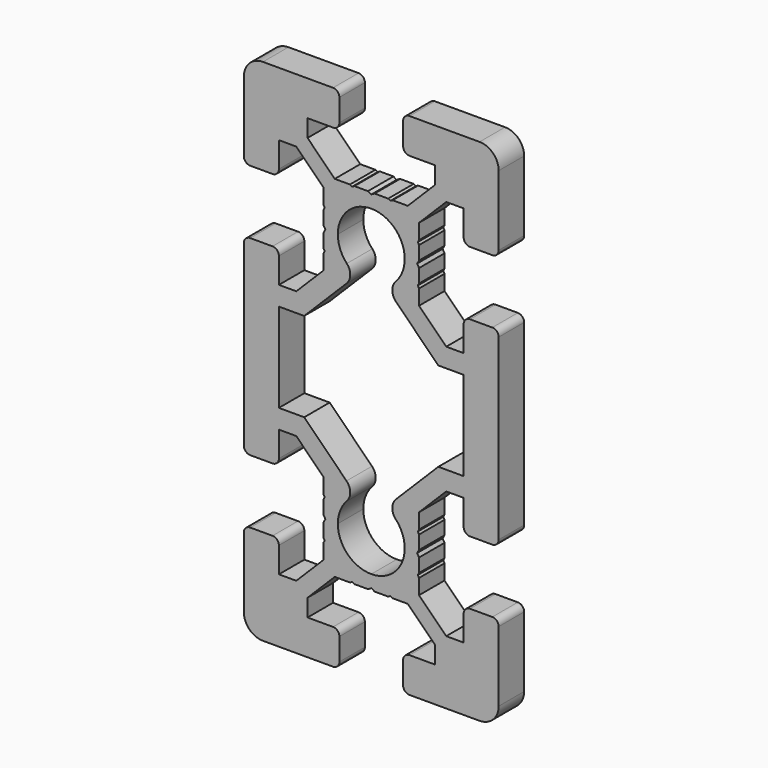
from build123d import *

# Parameters (mm, degrees)
F2_DEPTH = 5


# Not quite as in the source:
# - ends of sketch curves that miss each other by under 0.0002 mm in the source are joined


with BuildPart() as f2:
    # F1 (on Front) → F2 (new body)
    with BuildSketch(Plane.XZ):
        with BuildLine():
            Line((-19.72619, -25.25), (-23.22619, -25.25))
            ThreePointArc((-23.22619, -25.25), (-23.9332967812, -25.5428932188), (-24.22619, -26.25))
            Line((-24.22619, -26.25), (-24.22619, -37.25))
            ThreePointArc((-24.22619, -37.25), (-23.3475103436, -39.3713203436), (-21.22619, -40.25))
            Line((-21.22619, -40.25), (-10.22619, -40.25))
            ThreePointArc((-10.22619, -40.25), (-9.5190832188, -39.9571067812), (-9.22619, -39.25))
            Line((-9.22619, -39.25), (-9.22619, -35.75))
            ThreePointArc((-9.22619, -35.75), (-9.5190832188, -35.0428932188), (-10.22619, -34.75))
            Line((-10.22619, -34.75), (-14.22619, -34.75))
            Line((-14.22619, -34.75), (-14.22619, -32.017775))
            Line((-14.22619, -32.017775), (-9.958438, -27.75))
            Line((-9.958438, -27.75), (-7.5726, -27.75))
            Line((-7.5726, -27.75), (-7.22619, -27.55))
            Line((-7.22619, -27.55), (-6.87978, -27.75))
            Line((-6.87978, -27.75), (-4.745805, -27.75))
            Line((-4.745805, -27.75), (-4.22619, -27.45))
            Line((-4.22619, -27.45), (-3.706575, -27.75))
            Line((-3.706575, -27.75), (-1.5726, -27.75))
            Line((-1.5726, -27.75), (-1.22619, -27.55))
            Line((-1.22619, -27.55), (-0.87978, -27.75))
            Line((-0.87978, -27.75), (1.506057, -27.75))
            Line((1.506057, -27.75), (5.77381, -32.017782))
            Line((5.77381, -32.017782), (5.77381, -34.75))
            Line((5.77381, -34.75), (1.77381, -34.75))
            ThreePointArc((1.77381, -34.75), (1.0667032188, -35.0428932188), (0.77381, -35.75))
            Line((0.77381, -35.75), (0.77381, -39.25))
            ThreePointArc((0.77381, -39.25), (1.0667032188, -39.9571067812), (1.77381, -40.25))
            Line((1.77381, -40.25), (12.77381, -40.25))
            ThreePointArc((12.77381, -40.25), (14.8951303436, -39.3713203436), (15.77381, -37.25))
            Line((15.77381, -37.25), (15.77381, -26.25))
            ThreePointArc((15.77381, -26.25), (15.4809167812, -25.5428932188), (14.77381, -25.25))
            Line((14.77381, -25.25), (11.27381, -25.25))
            ThreePointArc((11.27381, -25.25), (10.5667032188, -25.5428932188), (10.27381, -26.25))
            Line((10.27381, -26.25), (10.27381, -30.25))
            Line((10.27381, -30.25), (7.541595, -30.25))
            Line((7.541595, -30.25), (3.27381, -25.98223))
            Line((3.27381, -25.98223), (3.27381, -23.59641))
            Line((3.27381, -23.59641), (3.07381, -23.25))
            Line((3.07381, -23.25), (3.27381, -22.90359))
            Line((3.27381, -22.90359), (3.27381, -20.769615))
            Line((3.27381, -20.769615), (2.97381, -20.25))
            Line((2.97381, -20.25), (3.27381, -19.730385))
            Line((3.27381, -19.730385), (3.27381, -17.59641))
            Line((3.27381, -17.59641), (3.07381, -17.25))
            Line((3.07381, -17.25), (3.27381, -16.90359))
            Line((3.27381, -16.90359), (3.27381, -14.517762))
            Line((3.27381, -14.517762), (7.541591, -10.25))
            Line((7.541591, -10.25), (10.27381, -10.25))
            Line((10.27381, -10.25), (10.27381, -14.25))
            ThreePointArc((10.27381, -14.25), (10.5667032188, -14.9571067812), (11.27381, -15.25))
            Line((11.27381, -15.25), (14.77381, -15.25))
            ThreePointArc((14.77381, -15.25), (15.4809167812, -14.9571067812), (15.77381, -14.25))
            Line((15.77381, -14.25), (15.77381, 13.75))
            ThreePointArc((15.77381, 13.75), (15.4809167812, 14.4571067812), (14.77381, 14.75))
            Line((14.77381, 14.75), (11.27381, 14.75))
            ThreePointArc((11.27381, 14.75), (10.5667032188, 14.4571067812), (10.27381, 13.75))
            Line((10.27381, 13.75), (10.27381, 9.75))
            Line((10.27381, 9.75), (7.541586, 9.75))
            Line((7.541586, 9.75), (3.27381, 14.01777))
            Line((3.27381, 14.01777), (3.27381, 16.40359))
            Line((3.27381, 16.40359), (3.07381, 16.75))
            Line((3.07381, 16.75), (3.27381, 17.09641))
            Line((3.27381, 17.09641), (3.27381, 19.230385))
            Line((3.27381, 19.230385), (2.97381, 19.75))
            Line((2.97381, 19.75), (3.27381, 20.269615))
            Line((3.27381, 20.269615), (3.27381, 22.40359))
            Line((3.27381, 22.40359), (3.07381, 22.75))
            Line((3.07381, 22.75), (3.27381, 23.09641))
            Line((3.27381, 23.09641), (3.27381, 25.482238))
            Line((3.27381, 25.482238), (7.541577, 29.75))
            Line((7.541577, 29.75), (10.27381, 29.75))
            Line((10.27381, 29.75), (10.27381, 25.75))
            ThreePointArc((10.27381, 25.75), (10.5667032188, 25.0428932188), (11.27381, 24.75))
            Line((11.27381, 24.75), (14.77381, 24.75))
            ThreePointArc((14.77381, 24.75), (15.4809167812, 25.0428932188), (15.77381, 25.75))
            Line((15.77381, 25.75), (15.77381, 36.75))
            ThreePointArc((15.77381, 36.75), (14.8951303436, 38.8713203436), (12.77381, 39.75))
            Line((12.77381, 39.75), (1.77381, 39.75))
            ThreePointArc((1.77381, 39.75), (1.0667032188, 39.4571067812), (0.77381, 38.75))
            Line((0.77381, 38.75), (0.77381, 35.25))
            ThreePointArc((0.77381, 35.25), (1.0667032188, 34.5428932188), (1.77381, 34.25))
            Line((1.77381, 34.25), (5.77381, 34.25))
            Line((5.77381, 34.25), (5.77381, 31.517777))
            Line((5.77381, 31.517777), (1.50604, 27.25))
            Line((1.50604, 27.25), (-0.87978, 27.25))
            Line((-0.87978, 27.25), (-1.22619, 27.05))
            Line((-1.22619, 27.05), (-1.5726, 27.25))
            Line((-1.5726, 27.25), (-3.706575, 27.25))
            Line((-3.706575, 27.25), (-4.22619, 26.95))
            Line((-4.22619, 26.95), (-4.745805, 27.25))
            Line((-4.745805, 27.25), (-6.87978, 27.25))
            Line((-6.87978, 27.25), (-7.22619, 27.05))
            Line((-7.22619, 27.05), (-7.5726, 27.25))
            Line((-7.5726, 27.25), (-9.958421, 27.25))
            Line((-9.958421, 27.25), (-14.22619, 31.517777))
            Line((-14.22619, 31.517777), (-14.22619, 34.25))
            Line((-14.22619, 34.25), (-10.22619, 34.25))
            ThreePointArc((-10.22619, 34.25), (-9.5190832188, 34.5428932188), (-9.22619, 35.25))
            Line((-9.22619, 35.25), (-9.22619, 38.75))
            ThreePointArc((-9.22619, 38.75), (-9.5190832188, 39.4571067812), (-10.22619, 39.75))
            Line((-10.22619, 39.75), (-21.22619, 39.75))
            ThreePointArc((-21.22619, 39.75), (-23.3475103436, 38.8713203436), (-24.22619, 36.75))
            Line((-24.22619, 36.75), (-24.22619, 25.75))
            ThreePointArc((-24.22619, 25.75), (-23.9332967812, 25.0428932188), (-23.22619, 24.75))
            Line((-23.22619, 24.75), (-19.72619, 24.75))
            ThreePointArc((-19.72619, 24.75), (-19.0190832188, 25.0428932188), (-18.72619, 25.75))
            Line((-18.72619, 25.75), (-18.72619, 29.75))
            Line((-18.72619, 29.75), (-15.993967, 29.75))
            Line((-15.993967, 29.75), (-11.72619, 25.482237))
            Line((-11.72619, 25.482237), (-11.72619, 23.09641))
            Line((-11.72619, 23.09641), (-11.52619, 22.75))
            Line((-11.52619, 22.75), (-11.72619, 22.40359))
            Line((-11.72619, 22.40359), (-11.72619, 20.269615))
            Line((-11.72619, 20.269615), (-11.42619, 19.75))
            Line((-11.42619, 19.75), (-11.72619, 19.230385))
            Line((-11.72619, 19.230385), (-11.72619, 17.09641))
            Line((-11.72619, 17.09641), (-11.52619, 16.75))
            Line((-11.52619, 16.75), (-11.72619, 16.40359))
            Line((-11.72619, 16.40359), (-11.72619, 14.017771))
            Line((-11.72619, 14.017771), (-15.993967, 9.75))
            Line((-15.993967, 9.75), (-18.72619, 9.75))
            Line((-18.72619, 9.75), (-18.72619, 13.75))
            ThreePointArc((-18.72619, 13.75), (-19.0190832188, 14.4571067812), (-19.72619, 14.75))
            Line((-19.72619, 14.75), (-23.22619, 14.75))
            ThreePointArc((-23.22619, 14.75), (-23.9332967812, 14.4571067812), (-24.22619, 13.75))
            Line((-24.22619, 13.75), (-24.22619, -14.25))
            ThreePointArc((-24.22619, -14.25), (-23.9332967812, -14.9571067812), (-23.22619, -15.25))
            Line((-23.22619, -15.25), (-19.72619, -15.25))
            ThreePointArc((-19.72619, -15.25), (-19.0190832188, -14.9571067812), (-18.72619, -14.25))
            Line((-18.72619, -14.25), (-18.72619, -10.25))
            Line((-18.72619, -10.25), (-15.993967, -10.25))
            Line((-15.993967, -10.25), (-11.72619, -14.517763))
            Line((-11.72619, -14.517763), (-11.72619, -16.90359))
            Line((-11.72619, -16.90359), (-11.52619, -17.25))
            Line((-11.52619, -17.25), (-11.72619, -17.59641))
            Line((-11.72619, -17.59641), (-11.72619, -19.730385))
            Line((-11.72619, -19.730385), (-11.42619, -20.25))
            Line((-11.42619, -20.25), (-11.72619, -20.769615))
            Line((-11.72619, -20.769615), (-11.72619, -22.90359))
            Line((-11.72619, -22.90359), (-11.52619, -23.25))
            Line((-11.52619, -23.25), (-11.72619, -23.59641))
            Line((-11.72619, -23.59641), (-11.72619, -25.982229))
            Line((-11.72619, -25.982229), (-15.993967, -30.25))
            Line((-15.993967, -30.25), (-18.72619, -30.25))
            Line((-18.72619, -30.25), (-18.72619, -26.25))
            ThreePointArc((-18.72619, -26.25), (-19.0190832188, -25.5428932188), (-19.72619, -25.25))
        make_face()
        with BuildLine():
            ThreePointArc((-8.0643043475, 16.1679086757), (-9.1104811627, 17.8248506973), (-9.47619, 19.75))
            ThreePointArc((-9.47619, 19.75), (-7.9385006012, 23.4623106012), (-4.22619, 25))
            ThreePointArc((-4.22619, 25), (-0.5138793988, 23.4623106012), (1.02381, 19.75))
            ThreePointArc((1.02381, 19.75), (0.6581010287, 17.8248503572), (-0.3880761513, 16.1679081412))
            ThreePointArc((-0.3880761513, 16.1679081412), (-0.9256396058, 14.768813042), (-0.3401495624, 13.3890874376))
            Line((-0.3401495624, 13.3890874376), (6.298947, 6.75))
            Line((6.298947, 6.75), (10.27381, 6.75))
            Line((10.27381, 6.75), (10.27381, -7.25))
            Line((10.27381, -7.25), (6.298954, -7.25))
            Line((6.298954, -7.25), (-0.340154, -13.889079))
            ThreePointArc((-0.340154, -13.889079), (-0.925646618, -15.2688067478), (-0.3880801087, -16.6679041014))
            ThreePointArc((-0.3880801087, -16.6679041014), (0.6580999921, -18.3248477273), (1.02381, -20.25))
            ThreePointArc((1.02381, -20.25), (-0.5138793988, -23.9623106012), (-4.22619, -25.5))
            ThreePointArc((-4.22619, -25.5), (-7.9385006012, -23.9623106012), (-9.47619, -20.25))
            ThreePointArc((-9.47619, -20.25), (-9.1104801262, -18.3248480674), (-8.0643004901, -16.6679045426))
            ThreePointArc((-8.0643004901, -16.6679045426), (-7.526735394, -15.2688080536), (-8.1122269376, -13.8890809376))
            Line((-8.1122269376, -13.8890809376), (-14.751329, -7.25))
            Line((-14.751329, -7.25), (-18.72619, -7.25))
            Line((-18.72619, -7.25), (-18.72619, 6.75))
            Line((-18.72619, 6.75), (-14.751328, 6.75))
            Line((-14.751328, 6.75), (-8.11223, 13.389088))
            ThreePointArc((-8.11223, 13.389088), (-7.5267403818, 14.768813761), (-8.0643043475, 16.1679086757))
        make_face(mode=Mode.SUBTRACT)
    extrude(amount=F2_DEPTH)


solid = f2.part
